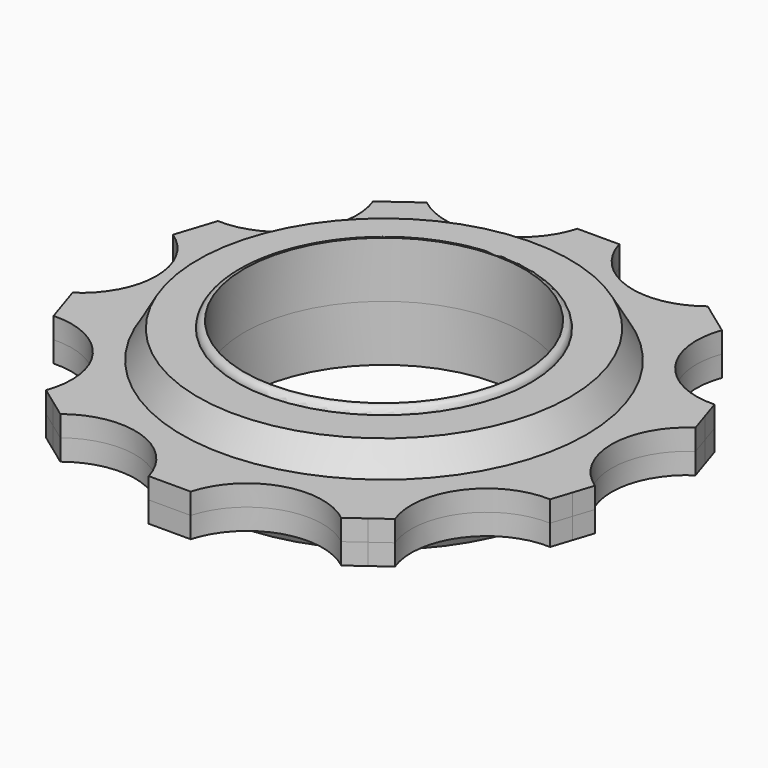
from build123d import *

# Parameters (mm, degrees)
F0_R     = 14.5
F1_DEPTH = 1.5
F0_R_2   = 10.5
F2_DEPTH = 3.5
F0_R_3   = 10
F3_DEPTH = 4
F5_R     = 0.49999


# Not quite as in the source:
# - a fillet or chamfer that OpenCascade refuses, or shapes differently, is made with other operations: its cross-section is extruded or revolved along the edge and cut away or added
# - a fillet or chamfer is up to 0.001 mm smaller than in the source, because OpenCascade refuses the exact size


with BuildPart() as f1:
    # F0 (on Top) → F1 (new body)
    with BuildSketch(Plane.XY):
        with BuildLine():
            Line((-17.7492067955, 7.3442602167), (-18.2127322871, 5.9176754423))
            Line((-18.2127322871, 5.9176754423), (-18.6762577786, 4.4910906678))
            ThreePointArc((-18.6762577786, 4.4910906678), (-16.275, 0), (-18.6762577786, -4.4910906678))
            Line((-18.6762577786, -4.4910906678), (-18.2127322871, -5.9176754423))
            Line((-18.2127322871, -5.9176754423), (-17.7492067955, -7.3442602167))
            ThreePointArc((-17.7492067955, -7.3442602167), (-13.1667515835, -9.5662049811), (-12.469613073, -14.6109975638))
            Line((-12.469613073, -14.6109975638), (-11.2560875814, -15.4926754423))
            Line((-11.2560875814, -15.4926754423), (-10.0425620898, -16.3743533207))
            ThreePointArc((-10.0425620898, -16.3743533207), (-5.0292515835, -15.4784448027), (-1.5, -19.15))
            Line((-1.5, -19.15), (0, -19.15))
            Line((0, -19.15), (1.5, -19.15))
            ThreePointArc((1.5, -19.15), (5.0292515835, -15.4784448027), (10.0425620898, -16.3743533207))
            Line((10.0425620898, -16.3743533207), (11.2560875814, -15.4926754423))
            Line((11.2560875814, -15.4926754423), (12.469613073, -14.6109975638))
            ThreePointArc((12.469613073, -14.6109975638), (13.1667515835, -9.5662049811), (17.7492067955, -7.3442602167))
            Line((17.7492067955, -7.3442602167), (18.2127322871, -5.9176754423))
            Line((18.2127322871, -5.9176754423), (18.6762577786, -4.4910906678))
            ThreePointArc((18.6762577786, -4.4910906678), (16.275, 0), (18.6762577786, 4.4910906678))
            Line((18.6762577786, 4.4910906678), (18.2127322871, 5.9176754423))
            Line((18.2127322871, 5.9176754423), (17.7492067955, 7.3442602167))
            ThreePointArc((17.7492067955, 7.3442602167), (13.1667515835, 9.5662049811), (12.469613073, 14.6109975638))
            Line((12.469613073, 14.6109975638), (11.2560875814, 15.4926754423))
            Line((11.2560875814, 15.4926754423), (10.0425620898, 16.3743533207))
            ThreePointArc((10.0425620898, 16.3743533207), (5.0292515835, 15.4784448027), (1.5, 19.15))
            Line((1.5, 19.15), (0, 19.15))
            Line((0, 19.15), (-1.5, 19.15))
            ThreePointArc((-1.5, 19.15), (-5.0292515835, 15.4784448027), (-10.0425620898, 16.3743533207))
            Line((-10.0425620898, 16.3743533207), (-11.2560875814, 15.4926754423))
            Line((-11.2560875814, 15.4926754423), (-12.469613073, 14.6109975638))
            ThreePointArc((-12.469613073, 14.6109975638), (-13.1667515835, 9.5662049811), (-17.7492067955, 7.3442602167))
        make_face()
        Circle(F0_R, mode=Mode.SUBTRACT)
    extrude(amount=F1_DEPTH)

    # F0 (on Top) → F2 (join)
    with BuildSketch(Plane.XY):
        Circle(F0_R)
        Circle(F0_R_2, mode=Mode.SUBTRACT)
    extrude(amount=F2_DEPTH)

    # F0 (on Top) → F3 (join)
    with BuildSketch(Plane.XY):
        Circle(F0_R_2)
        Circle(F0_R_3, mode=Mode.SUBTRACT)
    extrude(amount=F3_DEPTH)

    # F4: chamfer of 1.2 x 2.0784609691 on 1 edges, made by hand


with BuildPart() as f4_tool2:
    # F4_s3 → F4_t4 (revolve)
    with BuildSketch(Plane.XZ):
        Polygon((14.5, 1.4215390309), (13.3, 3.5), (14.5, 3.5), align=None)
    revolve(axis=Axis((0, 0, 3.5), (0, 0, 1)))

    split(bisect_by=Plane.XY.offset(1.5), keep=Keep.TOP)


with BuildPart() as f1_1:
    add(f1.part)

    # F4_t1: cut F4_tool2
    add(f4_tool2.part, mode=Mode.SUBTRACT)

    # F5 (radius 0.5 in the source; OpenCascade refuses exactly that, so slightly less here)
    f5_edges = [f1_1.edges().sort_by_distance(p)[0] for p in [
        (-10.5, 0, 4),
    ]]
    fillet(f5_edges, radius=F5_R)

    # F6: F1 across face


with BuildPart() as f1_2:
    add(f1_1.part)
    add(f1_1.part.mirror(Plane(origin=(0, 0, 0), x_dir=(1, 0, 0), z_dir=(0, 0, -1))))


solid = f1_2.part
